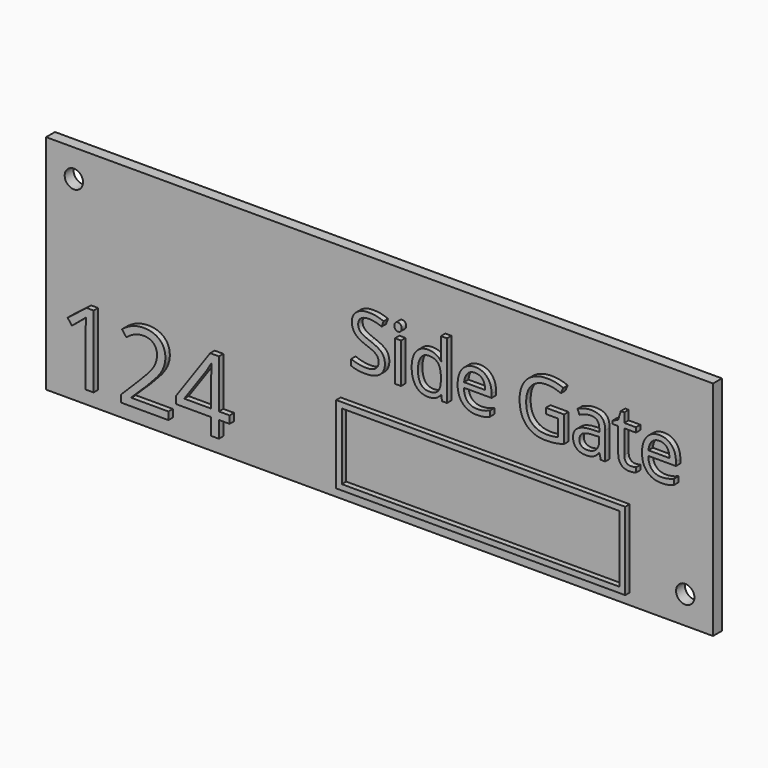
from build123d import *

# Parameters (mm, degrees)
F0_W         = 120
F0_H         = 40
F1_DEPTH     = 2
F3_D         = 3.3
F4_TEXT_SIZE = 13.4945178521
F5_DEPTH     = 1
F6_TEXT_SIZE = 18.1818181818
F7_DEPTH     = 1
F8_W         = 52
F8_H         = 14
F8_W_2       = 49.99999962
F8_H_2       = 11.99999962
F9_DEPTH     = 1


# Not quite as in the source:
# - Text() gives the source's letters only with a copy of the font that has no kerning and outlines rounded to 1/6400 em; it was checked with that copy


with BuildPart() as f1:
    # F0 (on Front) → F1 (new body)
    with BuildSketch(Plane.XZ):
        Rectangle(F0_W, F0_H)
    extrude(amount=F1_DEPTH)

    # F3 (through all)
    with Locations(Plane.XZ.offset(2)):
        with Locations((-55, 15), (55, -15)):
            Hole(F3_D / 2)

    # F4 (on face) → F5 (join)
    with BuildSketch(Plane.XZ.offset(2)):
        with Locations((-5, 2)):
            Text('Side Gate', F4_TEXT_SIZE, font='Open Sans', text_align=(TextAlign.LEFT, TextAlign.BOTTOM))
    extrude(amount=F5_DEPTH)

    # F6 (on face) → F7 (join)
    with BuildSketch(Plane.XZ.offset(2)):
        with Locations((-57, -17)):
            Text('124', F6_TEXT_SIZE, font='Open Sans', text_align=(TextAlign.LEFT, TextAlign.BOTTOM))
    extrude(amount=F7_DEPTH)

    # F8 (on face) → F9 (join)
    with BuildSketch(Plane.XZ.offset(2)):
        with Locations((19, -11)):
            Rectangle(F8_W, F8_H)
        with Locations((19, -11)):
            Rectangle(F8_W_2, F8_H_2, mode=Mode.SUBTRACT)
    extrude(amount=F9_DEPTH)


solid = f1.part
